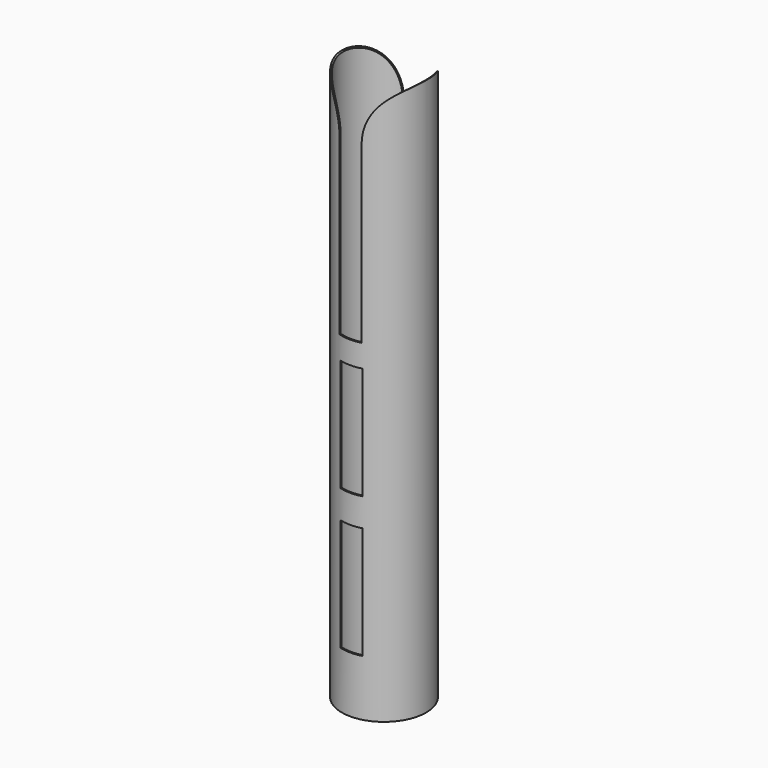
from build123d import *

# Parameters (mm, degrees)
F0_R        = 19.05
F1_DEPTH    = 254
F2_T        = -0.635
F3_W        = 10.16
F3_H        = 50.8
F3_H_2      = 127
F4_DEPTH    = 38.1
F5_T1_DEPTH = 127.6645661416
F5_T3_DEPTH = 127.6553906563
F5_T5_DEPTH = 127.6553906563
F5_T7_DEPTH = 127.6645661416


# Not quite as in the source:
# - a fillet or chamfer that OpenCascade refuses, or shapes differently, is made with other operations: its cross-section is extruded or revolved along the edge and cut away or added


with BuildPart() as f1:
    # F0 (on Top) → F1 (new body)
    with BuildSketch(Plane.XY):
        Circle(F0_R)
    extrude(amount=F1_DEPTH)

    # F2
    f2_openings = [f1.faces().sort_by_distance(p)[0] for p in [
        (0, 0, 0),
        (0, 0, 254),
    ]]
    offset(amount=F2_T, openings=f2_openings)

    # F3 (on Front) → F4 (cut, symmetric)
    with BuildSketch(Plane.XZ):
        with Locations((0, 50.8)):
            Rectangle(F3_W, F3_H)
        with Locations((-3.17e-08, 114.3)):
            Rectangle(F3_W, F3_H)
        with Locations((-0.4444076066, 213.36)):
            Rectangle(F3_W, F3_H_2)
    extrude(amount=F4_DEPTH, both=True, mode=Mode.SUBTRACT)

    # F5: fillet of radius 25.4 on 4 edges, made by hand

    # F5_s2 → F5_t1 (cut)
    with BuildSketch(Plane.XZ.offset(-45.9331805498)):
        with BuildLine():
            ThreePointArc((-5.5244076066, 228.6), (-12.9638953644, 246.5605122421), (-30.9244076066, 254))
            Line((-30.9244076066, 254), (-5.5244076066, 254))
            Line((-5.5244076066, 254), (-5.5244076066, 228.6))
        make_face()
    extrude(amount=F5_T1_DEPTH, mode=Mode.SUBTRACT)

    # F5_s4 → F5_t3 (cut)
    with BuildSketch(Plane.XZ.offset(-45.6780049332)):
        with BuildLine():
            ThreePointArc((30.0355923934, 254), (12.0750801513, 246.5605122421), (4.6355923934, 228.6))
            Line((4.6355923934, 228.6), (4.6355923934, 254))
            Line((4.6355923934, 254), (30.0355923934, 254))
        make_face()
    extrude(amount=F5_T3_DEPTH, mode=Mode.SUBTRACT)

    # F5_s6 → F5_t5 (cut)
    with BuildSketch(Plane.XZ.offset(-81.9773857231)):
        with BuildLine():
            ThreePointArc((30.0355923934, 254), (12.0750801513, 246.5605122421), (4.6355923934, 228.6))
            Line((4.6355923934, 228.6), (4.6355923934, 254))
            Line((4.6355923934, 254), (30.0355923934, 254))
        make_face()
    extrude(amount=F5_T5_DEPTH, mode=Mode.SUBTRACT)

    # F5_s8 → F5_t7 (cut)
    with BuildSketch(Plane.XZ.offset(-81.7313855918)):
        with BuildLine():
            ThreePointArc((-30.9244076066, 254), (-12.9638953644, 246.5605122421), (-5.5244076066, 228.6))
            Line((-5.5244076066, 228.6), (-5.5244076066, 254))
            Line((-5.5244076066, 254), (-30.9244076066, 254))
        make_face()
    extrude(amount=F5_T7_DEPTH, mode=Mode.SUBTRACT)


solid = f1.part
